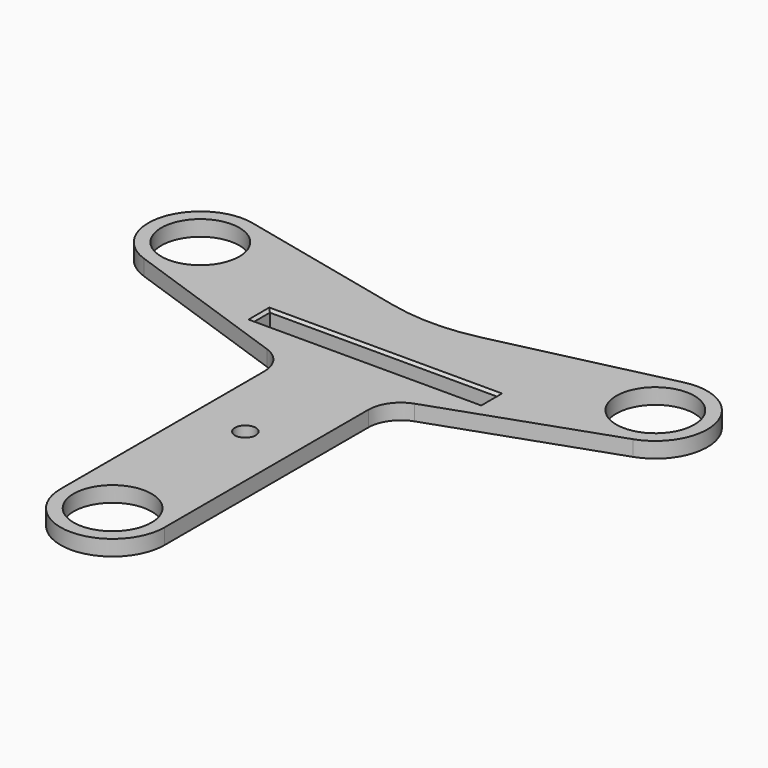
from build123d import *

# Parameters (mm, degrees)
F0_R     = 6
F0_R_2   = 1.6
F0_W     = 35
F0_H     = 3.2
F1_DEPTH = 2.4
F2_SIZE  = 0.4
F3_R     = 30
F4_R     = 5


with BuildPart() as f1:
    # F0 (on Top) → F1 (new body)
    with BuildSketch(Plane.XY):
        with BuildLine():
            Line((-8.000963252, 2.3046399066), (-8, -40.4145188433))
            ThreePointArc((-8, -40.4145188433), (0, -48.4145188433), (8, -40.4145188433))
            Line((8, -40.4145188433), (7.9974217916, 2.303660399))
            Line((7.9974217916, 2.303660399), (37.6375477343, 12.6545551411))
            ThreePointArc((37.6375477343, 12.6545551411), (42.6856959969, 22.427637102), (33.2034437111, 28.002923954))
            Line((33.2034437111, 28.002923954), (-0.0031576851, 20.3502692862))
            Line((-0.0031576851, 20.3502692862), (-33.2031192071, 28.002849163))
            ThreePointArc((-33.2031192071, 28.002849163), (-42.6856411927, 22.4278267944), (-37.6376061638, 12.654575546))
            Line((-37.6376061638, 12.654575546), (-8.000963252, 2.3046399066))
        make_face()
        with Locations((0, -40.4145188433)):
            Circle(F0_R, mode=Mode.SUBTRACT)
        with Locations((0, -14.8963702892)):
            Circle(F0_R_2, mode=Mode.SUBTRACT)
        with Locations((-35, 20.2072594216)):
            Circle(F0_R, mode=Mode.SUBTRACT)
        with Locations((0, 10.1036297108)):
            Rectangle(F0_W, F0_H, mode=Mode.SUBTRACT)
        with Locations((35, 20.2072594216)):
            Circle(F0_R, mode=Mode.SUBTRACT)
    extrude(amount=F1_DEPTH)

    # F2
    f2_edges = [f1.edges().sort_by_distance(p)[0] for p in [
        (-17.5, 10.10363, 2.4),
        (0, 11.70363, 2.4),
        (0, 8.50363, 2.4),
        (17.5, 10.10363, 2.4),
    ]]
    chamfer(f2_edges, length=F2_SIZE)

    # F3
    f3_edges = [f1.edges().sort_by_distance(p)[0] for p in [
        (-0.003158, 20.350269, 1.2),
    ]]
    fillet(f3_edges, radius=F3_R)

    # F4
    f4_edges = [f1.edges().sort_by_distance(p)[0] for p in [
        (7.997422, 2.30366, 1.2),
        (-8.000963, 2.30464, 1.2),
    ]]
    fillet(f4_edges, radius=F4_R)


solid = f1.part
